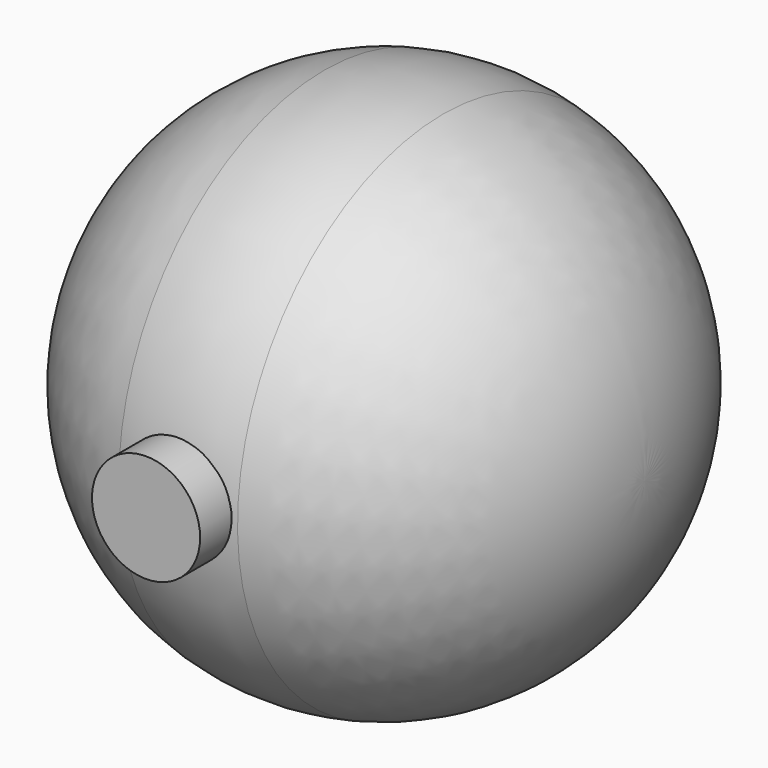
from build123d import *

# Parameters (mm, degrees)
F2_R     = 4.6179703718
F3_DEPTH = 25.4


with BuildPart() as f1:
    # F0 (on Front) → F1 (revolve)
    with BuildSketch(Plane.XZ):
        with BuildLine():
            Line((27.3387702071, 0), (44.5344567494, 0))
            ThreePointArc((44.5344567494, 0), (39.8057351852, 14.01585605), (27.3387702071, 21.9769999804))
            Line((27.3387702071, 21.9769999804), (27.3387702071, 0))
        make_face()
    revolve(axis=Axis((22.2672283747, 0, 0), (1, 0, 0)))


with BuildPart() as f1b:
    # F0 (on Front) → F1, piece 2 (revolve)
    with BuildSketch(Plane.XZ):
        with BuildLine():
            Line((17.1956865423, 21.9769999804), (27.3387702071, 21.9769999804))
            ThreePointArc((27.3387702071, 21.9769999804), (22.2672283747, 22.5621809582), (17.1956865423, 21.9769999804))
        make_face()
    revolve(axis=Axis((22.2672283747, 0, 0), (1, 0, 0)))


with BuildPart() as f1c:
    # F0 (on Front) → F1, piece 3 (revolve)
    with BuildSketch(Plane.XZ):
        with BuildLine():
            Line((17.1956865423, 0), (17.1956865423, 21.9769999804))
            ThreePointArc((17.1956865423, 21.9769999804), (4.7287215641, 14.01585605), (0, 0))
            Line((0, 0), (17.1956865423, 0))
        make_face()
    revolve(axis=Axis((22.2672283747, 0, 0), (1, 0, 0)))


with BuildPart() as f3:
    # F2 (on Front) → F3 (new body)
    with BuildSketch(Plane.XZ):
        with Locations((22.2672283747, 0.2930246443)):
            Circle(F2_R)
    extrude(amount=F3_DEPTH)


solid = Compound([f1.part, f1b.part, f1c.part, f3.part])
